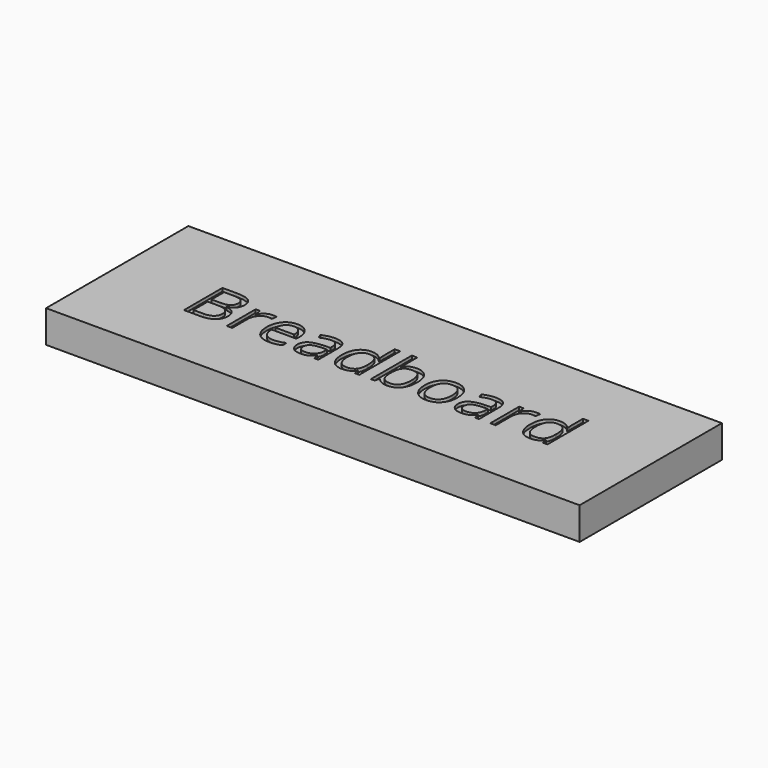
from build123d import *

# Parameters (mm, degrees)
F0_W         = 165
F0_H         = 55
F1_DEPTH     = 10
F2_TEXT_SIZE = 20.8333333333
F3_DEPTH     = 1


# Not quite as in the source:
# - Text() gives the source's letters only with a copy of the font that has no kerning and outlines rounded to 1/6400 em; it was checked with that copy


with BuildPart() as f1:
    # F0 (on Top) → F1 (new body)
    with BuildSketch(Plane.XY):
        Rectangle(F0_W, F0_H)
    extrude(amount=F1_DEPTH)

    # F2 (on face) → F3 (cut)
    with BuildSketch(Plane.XY.offset(10)):
        with Locations((-57.9085286458, -7.5)):
            Text('Breadboard', F2_TEXT_SIZE, font='Open Sans', text_align=(TextAlign.LEFT, TextAlign.BOTTOM))
    extrude(amount=-F3_DEPTH, mode=Mode.SUBTRACT)


solid = f1.part
